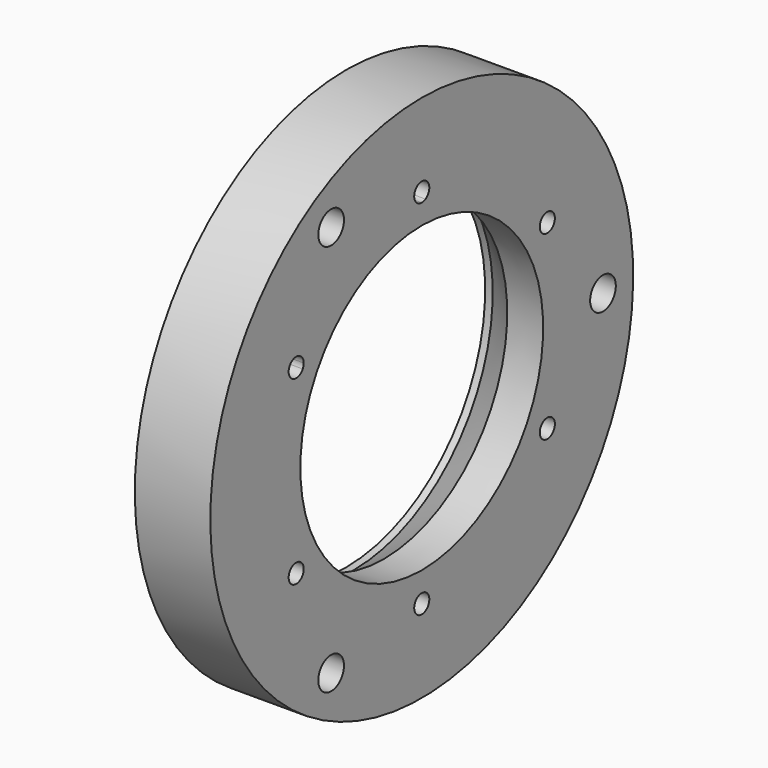
from build123d import *

# Parameters (mm, degrees)
F2_R            = 4.25
F3_DEPTH        = 20.001
F3_COPIES_COUNT = 3
F5_DEPTH        = 15
F5_COPIES_COUNT = 6


# Not quite as in the source:
# - a fillet or chamfer that OpenCascade refuses, or shapes differently, is made with other operations: its cross-section is extruded or revolved along the edge and cut away or added
# - a pattern or mirror of a feature is missing from the dataset's text; its kind, count and spacing are read off the source's solid


with BuildPart() as f1:
    # F0 (on Front) → F1 (revolve)
    with BuildSketch(Plane.XZ):
        Polygon((-10, 40.8116262015), (0, 40.2), (0, 70), (-20, 70), (-20, 46), (-18, 46), align=None)
    revolve(axis=Axis((12.3917190358, 0, 0), (1, 0, 0)))

    # F2 (on face) → F3 (cut, through all)
    with BuildSketch(Plane(origin=(-20, 0, 0), x_dir=(0, -1, 0), z_dir=(-1, 0, 0))):
        with Locations((-60, 0)):
            Circle(F2_R)
    f3 = extrude(amount=-F3_DEPTH, mode=Mode.SUBTRACT)

    # F3_copies: F3 ×3 about axis
    f3_copies_axis = Axis((0, 0, 0), (1, 0, 0))
    for i in range(1, F3_COPIES_COUNT):
        add(f3.rotate(f3_copies_axis, i * 360 / F3_COPIES_COUNT), mode=Mode.SUBTRACT)

    # F4 (on face) → F5 (cut)
    with BuildSketch(Plane.YZ):
        with BuildLine():
            ThreePointArc((-39.0692193817, 24), (-43.9840339474, 24.6470476128), (-39.4041558722, 22.75))
            ThreePointArc((-39.4041558722, 22.75), (-39.1544048159, 23.3529523872), (-39.0692193817, 24))
        make_face()
    f5 = extrude(amount=-F5_DEPTH, mode=Mode.SUBTRACT)

    # F5_copies: F5 ×6 about axis
    f5_copies_axis = Axis((0, 0, 0), (1, 0, 0))
    for i in range(1, F5_COPIES_COUNT):
        add(f5.rotate(f5_copies_axis, i * 360 / F5_COPIES_COUNT), mode=Mode.SUBTRACT)

    # F6: chamfer of 2.5 x 1.5021515476 on 6 edges, made by hand

    # F6_s1 → F6_t2 (revolve)
    with BuildSketch(Plane(origin=(0, 0, 0), x_dir=(1, 0, 0), z_dir=(0, -0.5, -0.8660254038))):
        Polygon((-13.4978484524, 45.5), (-15, 48), (-15, 45.5), align=None)
    revolve(axis=Axis((-15, -41.5692193817, 24), (1, 0, 0)))

    # F6_s3 → F6_t4 (revolve)
    with BuildSketch(Plane(origin=(0, 0, 0), x_dir=(1, 0, 0), z_dir=(0, -0.5, 0.8660254038))):
        Polygon((-13.4978484524, 45.5), (-15, 48), (-15, 45.5), align=None)
    revolve(axis=Axis((-15, 41.5692193817, 24), (1, 0, 0)))

    # F6_s5 → F6_t6 (revolve)
    with BuildSketch(Plane(origin=(0, 0, 0), x_dir=(1, 0, 0), z_dir=(0, 0.5, 0.8660254038))):
        Polygon((-13.4978484524, 45.5), (-15, 48), (-15, 45.5), align=None)
    revolve(axis=Axis((-15, 41.5692193817, -24), (1, 0, 0)))

    # F6_s7 → F6_t8 (revolve)
    with BuildSketch(Plane.XZ):
        Polygon((-13.4978484524, 45.5), (-15, 48), (-15, 45.5), align=None)
    revolve(axis=Axis((-15, 0, 48), (1, 0, 0)))

    # F6_s9 → F6_t10 (revolve)
    with BuildSketch(Plane.XZ):
        Polygon((-13.4978484524, -45.5), (-15, -48), (-15, -45.5), align=None)
    revolve(axis=Axis((-15, 0, -48), (1, 0, 0)))

    # F6_s11 → F6_t12 (revolve)
    with BuildSketch(Plane(origin=(0, 0, 0), x_dir=(1, 0, 0), z_dir=(0, 0.5, -0.8660254038))):
        Polygon((-13.4978484524, 45.5), (-15, 48), (-15, 45.5), align=None)
    revolve(axis=Axis((-15, -41.5692193817, -24), (1, 0, 0)))


solid = f1.part
